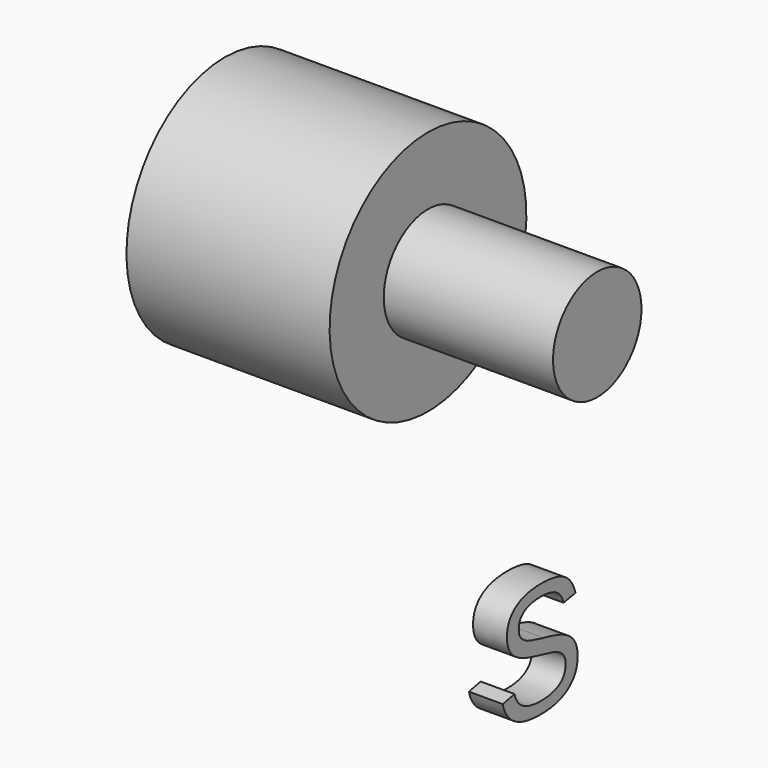
from build123d import *

# Parameters (mm, degrees)
F0_W         = 30
F0_H         = 10
F2_R         = 8.1642217342
F3_DEPTH     = 25
F4_TEXT_SIZE = 24.0036286414
F5_DEPTH     = 5


# Not quite as in the source:
# - Text() gives the source's letters only with a copy of the font that has no kerning and outlines rounded to 1/6400 em; it was checked with that copy


with BuildPart() as f1:
    # F0 (on Front) → F1 (revolve)
    with BuildSketch(Plane.XZ):
        with Locations((-22.6480278652, 17.7530375835)):
            Rectangle(F0_W, F0_H)
    revolve(axis=Axis((-22.2039490473, 0, 4.5888158493), (1, 0, 0)))


with BuildPart() as f3:
    # F2 (on face) → F3 (new body)
    with BuildSketch(Plane.YZ.offset(-7.6480278652)):
        with Locations((0, 4.5888158493)):
            Circle(F2_R)
    extrude(amount=F3_DEPTH)


with BuildPart() as f5:
    # F4 (on Right) → F5 (new body)
    with BuildSketch(Plane.YZ):
        with Locations((-3.0991747044, -50.6354644895)):
            Text('S', F4_TEXT_SIZE, font='Arimo', text_align=(TextAlign.LEFT, TextAlign.BOTTOM))
    extrude(amount=F5_DEPTH)


solid = Compound([f1.part, f3.part, f5.part])
